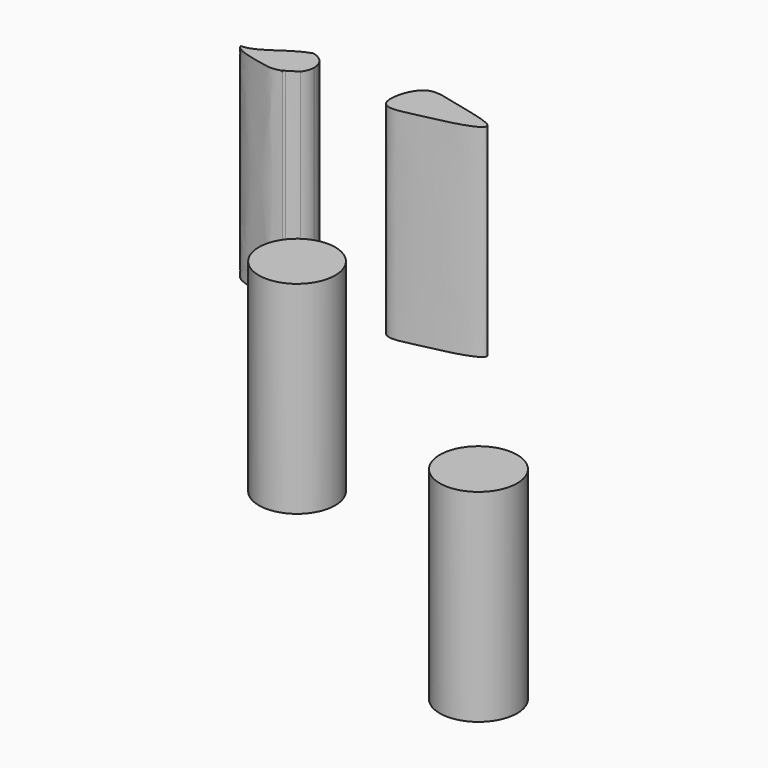
from build123d import *

# Parameters (mm, degrees)
F1_DEPTH = 25.4
F0_R     = 4.849575774
F0_R_2   = 4.7910280634


with BuildPart() as f1:
    # F0 (on Top) → F1 (new body)
    with BuildSketch(Plane.XY):
        with BuildLine():
            add(Edge.make_bspline(
                [(-36.629460752, 38.306619972), (-35.2596026769, 38.337745191), (-33.9741809776, 39.3643837081), (-32.5749787872, 40.2901070833)],
                knots=[0.6268692611, 0.6268692611, 0.6268692611, 0.6268692611, 0.6903877561, 0.6903877561, 0.6903877561, 0.6903877561], degree=3))
            add(Edge.make_bspline(
                [(-36.629460752, 38.306619972), (-36.5009242652, 37.5147103232), (-32.4045597695, 36.6803890088), (-31.3956164861, 36.4137841195), (-30.1884636283, 36.7730483413)],
                knots=[0.4052207067, 0.4052207067, 0.4052207067, 0.4052207067, 0.5540707536, 0.6779215323, 0.6779215323, 0.6779215323, 0.6779215323], degree=3))
            add(Edge.make_bspline(
                [(-29.9405695443, 36.9576867972), (-30.0242676146, 36.8975228318), (-30.1069616711, 36.8359980864), (-30.1884636283, 36.7730483413)],
                knots=[0.9111567917, 0.9111567917, 0.9111567917, 0.9111567917, 0.914558566, 0.914558566, 0.914558566, 0.914558566], degree=3))
            ThreePointArc((-29.9405695443, 36.9576867972), (-32.3276105514, 37.7781492192), (-32.5749787872, 40.2901070833))
        make_face()
        with BuildLine():
            add(Edge.make_bspline(
                [(-32.5749787872, 40.2901070833), (-31.8115797284, 40.7951780146), (-31.0143110677, 41.2702090361), (-30.1509803545, 41.5371289323)],
                knots=[0.6903877561, 0.6903877561, 0.6903877561, 0.6903877561, 0.7250431902, 0.7250431902, 0.7250431902, 0.7250431902], degree=3))
            ThreePointArc((-32.5749787872, 40.2901070833), (-32.3276105514, 37.7781492192), (-29.9405695443, 36.9576867972))
            add(Edge.make_bspline(
                [(-28.7036776433, 37.7278240007), (-29.1251753541, 37.4970904356), (-29.544134633, 37.2426527017), (-29.9405695443, 36.9576867972)],
                knots=[0.895044328, 0.895044328, 0.895044328, 0.895044328, 0.9111567917, 0.9111567917, 0.9111567917, 0.9111567917], degree=3))
            ThreePointArc((-28.7036776433, 37.7278240007), (-28.2996155266, 38.4293974522), (-28.1593097707, 39.2267592251))
            ThreePointArc((-28.1593097707, 39.2267592251), (-28.7259577315, 40.7519280599), (-30.1509803545, 41.5371289323))
        make_face()
    extrude(amount=F1_DEPTH)


with BuildPart() as f1b:
    # F0 (on Top) → F1, piece 2 (new body)
    with BuildSketch(Plane.XY):
        with BuildLine():
            add(Edge.make_bspline(
                [(-16.9997550547, 41.9871881604), (-16.0219392875, 42.9402709042), (-13.0614260868, 41.9290089772), (-5.5003551978, 40.4668337919), (-9.4821227835, 38.5765156015), (-13.5479301269, 37.8724685241), (-19.1404792258, 36.3043489214), (-17.9886072852, 41.0233481114), (-16.9997550547, 41.9871881604)],
                knots=[0, 0, 0, 0, 0.1682898556, 0.3642056637, 0.4849856044, 0.6676425216, 0.8298106815, 1, 1, 1, 1], degree=3))
        make_face()
    extrude(amount=F1_DEPTH)


with BuildPart() as f1c:
    # F0 (on Top) → F1, piece 3 (new body)
    with BuildSketch(Plane.XY):
        with Locations((37.5953651965, -17.2086451203)):
            Circle(F0_R)
    extrude(amount=F1_DEPTH)


with BuildPart() as f1d:
    # F0 (on Top) → F1, piece 4 (new body)
    with BuildSketch(Plane.XY):
        with Locations((-3.8110457826, 6.1016320251)):
            Circle(F0_R_2)
    extrude(amount=F1_DEPTH)


solid = Compound([f1.part, f1b.part, f1c.part, f1d.part])
